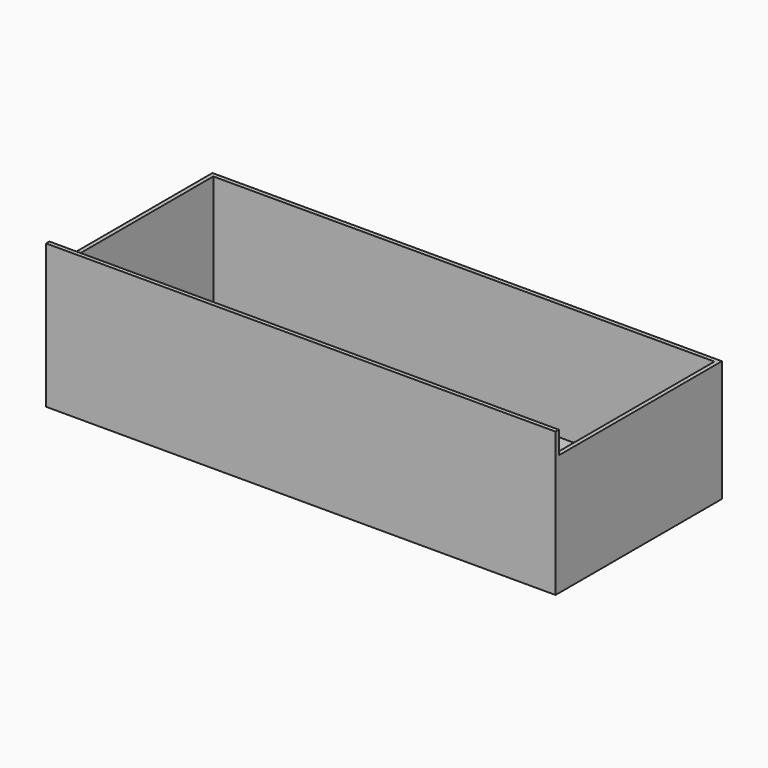
from build123d import *

# Parameters (mm, degrees)
F0_W     = 147
F0_H     = 60
F1_DEPTH = 35
F2_W     = 147
F2_H     = 1.6
F3_DEPTH = 6.5
F4_T     = -1.2
F5_DEPTH = 0.4


# Not quite as in the source:
# - a shell that OpenCascade refuses in one call is made with other operations: the cavity is built on its own and cut out


with BuildPart() as f1:
    # F0 (on Top) → F1 (new body)
    with BuildSketch(Plane.XY):
        with Locations((2.3024454713, -14.3951082311)):
            Rectangle(F0_W, F0_H)
    extrude(amount=F1_DEPTH)

    # F2 (on face) → F3 (join)
    with BuildSketch(Plane.XY.offset(35)):
        with Locations((2.3024454713, -43.5951082311)):
            Rectangle(F2_W, F2_H)
    extrude(amount=F3_DEPTH)

    # F4: a shell. OpenCascade refuses it in one call, so the cavity is built on its own and cut out:
    # the body offset inwards by the wall thickness, plus a prism from it out through each open face.
    f4_core = offset(f1.part, amount=F4_T, kind=Kind.INTERSECTION, mode=Mode.PRIVATE)
    f4_exits = [f4_core.faces().sort_by_distance(p)[0] for p in [
        (2.302445, -14.395108, 33.8),
    ]]
    add(f4_core, mode=Mode.SUBTRACT)
    extrude(f4_exits, amount=-F4_T, mode=Mode.SUBTRACT)

    # F5 (cut): a face of the model
    f5_faces = [f1.faces().sort_by_distance(p)[0] for p in [
        (2.3024454713, -42.7951082311, 38.25),
    ]]
    extrude(f5_faces, amount=-F5_DEPTH, mode=Mode.SUBTRACT)


solid = f1.part
